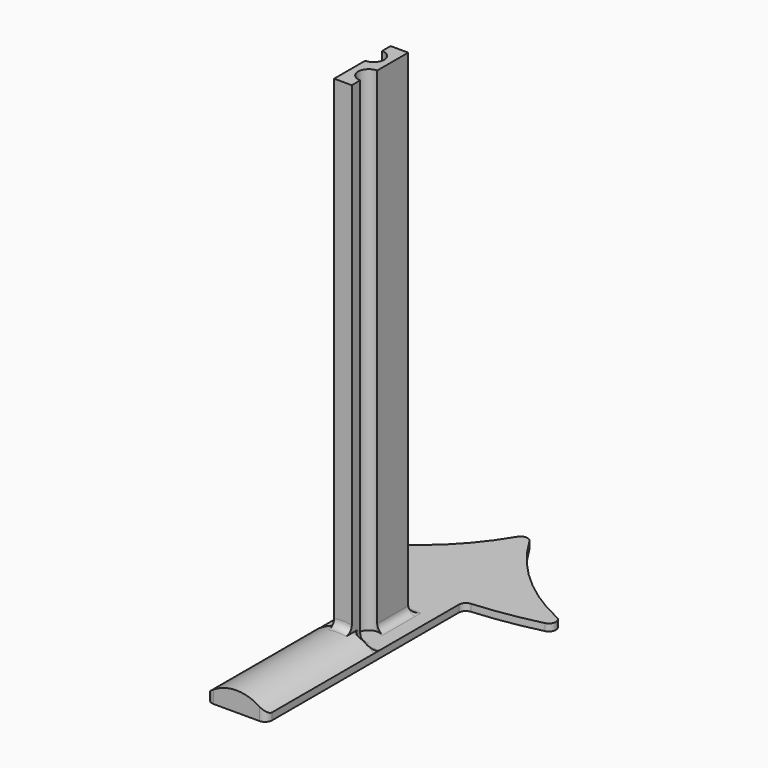
from build123d import *

# Parameters (mm, degrees)
F1_DEPTH      = 2
F3_DEPTH      = 140
F5_DEPTH      = 38
F6_S2_W       = 2
F6_S2_H       = 2
F6_T3_DEPTH   = 2
F6_S7_W       = 2
F6_S7_H       = 2
F6_T8_DEPTH   = 2
F6_T13_DEPTH  = 16
F6_S14_R      = 3
F6_T15_DEPTH  = 10
F6_T18_DEPTH  = 8
F6_S19_R      = 3
F6_T20_DEPTH  = 6
F6_T23_DEPTH  = 5
F6_T26_DEPTH  = 2
F6_T29_DEPTH  = 2
F6_T32_DEPTH  = 6.2698148841
F6_S33_R      = 12
F6_T34_DEPTH  = 5
F6_T37_DEPTH  = 4.0036432176
F6_S38_R      = 12
F6_T39_DEPTH  = 4
F6_T42_DEPTH  = 6.2698148841
F6_S43_R      = 12
F6_T44_DEPTH  = 5
F6_T47_DEPTH  = 4.0036432176
F6_S48_R      = 12
F6_T49_DEPTH  = 4
F6_T52_DEPTH  = 13.7211477996
F6_S53_R      = 3
F6_T54_DEPTH  = 9
F6_T57_DEPTH  = 5.7211477996
F6_S58_R      = 3
F6_T59_DEPTH  = 5
F6_T62_ANGLE  = 71.7972504735
F6_T68_DEPTH  = 21
F6_T72_DEPTH  = 10
F6_T78_DEPTH  = 10
F6_T82_DEPTH  = 13
F6_T88_DEPTH  = 12
F6_T91_DEPTH  = 12
F6_T94_DEPTH  = 32.0377713688
F6_T97_DEPTH  = 32.0377713688
F6_T100_DEPTH = 19.7312172526


# Not quite as in the source:
# - a fillet or chamfer that OpenCascade refuses, or shapes differently, is made with other operations: its cross-section is extruded or revolved along the edge and cut away or added


with BuildPart() as f1:
    # F0 (on Top) → F1 (new body)
    with BuildSketch(Plane.XY):
        with BuildLine():
            ThreePointArc((-34.7443990516, -30.0072931229), (-21.7619757905, -33.1321767709), (-8.5036432176, -34.7211477996))
            Line((-8.5036432176, -34.7211477996), (-8.5036432176, -104.7211477996))
            Line((-8.5036432176, -104.7211477996), (0, -104.7211477996))
            Line((0, -104.7211477996), (8.5036432176, -104.7211477996))
            Line((8.5036432176, -104.7211477996), (8.5036432176, -34.7211477996))
            ThreePointArc((8.5036432176, -34.7211477996), (21.7619757905, -33.1321767709), (34.7443990516, -30.0072931229))
            ThreePointArc((34.7443990516, -30.0072931229), (14.4817817228, -18.350360614), (0, 0))
            ThreePointArc((0, 0), (-14.4817817228, -18.350360614), (-34.7443990516, -30.0072931229))
        make_face()
    extrude(amount=F1_DEPTH)

    # F2 (on face) → F3 (join)
    with BuildSketch(Plane.XY.offset(2)):
        with BuildLine():
            Line((-2.5, -67), (2.5, -67))
            Line((2.5, -67), (2.5, -64))
            ThreePointArc((2.5, -64), (-0.5, -61), (2.5, -58))
            Line((2.5, -58), (2.5, -47))
            Line((2.5, -47), (-2.5, -47))
            Line((-2.5, -47), (-2.5, -50))
            ThreePointArc((-2.5, -50), (0.5, -53), (-2.5, -56))
            Line((-2.5, -56), (-2.5, -67))
        make_face()
    extrude(amount=F3_DEPTH)

    # F4 (on face) → F5 (join)
    with BuildSketch(Plane.XZ.offset(104.7211477996)):
        with BuildLine():
            ThreePointArc((8.5036432176, 2), (0, 5.5331202898), (-8.5036432176, 2))
            Line((-8.5036432176, 2), (8.5036432176, 2))
        make_face()
    extrude(amount=-F5_DEPTH)

    # F6: fillet of radius 2 on 17 edges, made by hand


with BuildPart() as f6_tool1:
    # F6_s2 → F6_t3 (new body)
    with BuildSketch(Plane.XZ.offset(64.7211477996)):
        with Locations((3.5, 3)):
            Rectangle(F6_S2_W, F6_S2_H)
    extrude(amount=F6_T3_DEPTH)

    # F6_s4 → F6_t5 (revolve, cut)
    with BuildSketch(Plane(origin=(4.5, -64.7211477996, 4), x_dir=(0.7071067812, 0, 0.7071067812), z_dir=(0.7071067812, 0, -0.7071067812))):
        with BuildLine():
            ThreePointArc((0, -2), (2, 0), (0, 2))
            Line((0, 2), (0, -2))
        make_face()
    revolve(axis=Axis((4.5, -64.7211477996, 4), (0, -1, 0)), mode=Mode.SUBTRACT)


with BuildPart() as f6_tool6:
    # F6_s7 → F6_t8 (new body)
    with BuildSketch(Plane.YZ.offset(-4.5)):
        with Locations((-65.7211477996, 3)):
            Rectangle(F6_S7_W, F6_S7_H)
    extrude(amount=F6_T8_DEPTH)

    # F6_s9 → F6_t10 (revolve, cut)
    with BuildSketch(Plane(origin=(-4.5, -64.7211477996, 4), x_dir=(0, 0.7071067812, 0.7071067812), z_dir=(0, 0.7071067812, -0.7071067812))):
        with BuildLine():
            ThreePointArc((0, -2), (2, 0), (0, 2))
            Line((0, 2), (0, -2))
        make_face()
    revolve(axis=Axis((-4.5, -64.7211477996, 4), (1, 0, 0)), mode=Mode.SUBTRACT)


with BuildPart() as f6_tool11:
    # F6_s12 → F6_t13 (new body)
    with BuildSketch(Plane.XZ.offset(63)):
        with BuildLine():
            ThreePointArc((4.5, 2), (3.0857864376, 2.5857864376), (2.5, 4))
            Line((2.5, 4), (2.5, 2))
            Line((2.5, 2), (4.5, 2))
        make_face()
    extrude(amount=-F6_T13_DEPTH)

    # F6_s14 → F6_t15 (cut, symmetric)
    with BuildSketch(Plane.XY.offset(3)):
        with Locations((2.5, -61)):
            Circle(F6_S14_R)
    extrude(amount=F6_T15_DEPTH, both=True, mode=Mode.SUBTRACT)


with BuildPart() as f6_tool16:
    # F6_s17 → F6_t18 (new body)
    with BuildSketch(Plane.XZ.offset(47)):
        with BuildLine():
            ThreePointArc((-4.5, 2), (-3.0857864376, 2.5857864376), (-2.5, 4))
            Line((-2.5, 4), (-2.5, 2))
            Line((-2.5, 2), (-4.5, 2))
        make_face()
    extrude(amount=F6_T18_DEPTH)

    # F6_s19 → F6_t20 (cut, symmetric)
    with BuildSketch(Plane.XY.offset(3)):
        with Locations((-2.5, -53)):
            Circle(F6_S19_R)
    extrude(amount=F6_T20_DEPTH, both=True, mode=Mode.SUBTRACT)


with BuildPart() as f6_tool21:
    # F6_s22 → F6_t23 (new body)
    with BuildSketch(Plane.YZ.offset(2.5)):
        with BuildLine():
            ThreePointArc((-45, 2), (-46.4142135624, 2.5857864376), (-47, 4))
            Line((-47, 4), (-47, 2))
            Line((-47, 2), (-45, 2))
        make_face()
    extrude(amount=-F6_T23_DEPTH)


with BuildPart() as f6_tool24:
    # F6_s25 → F6_t26 (new body)
    with BuildSketch(Plane.XY):
        with BuildLine():
            ThreePointArc((-10.349778168, -34.5937272007), (-9.0360380086, -35.2290743164), (-8.5036432176, -36.5877998039))
            Line((-8.5036432176, -36.5877998039), (-8.5036432176, -34.7211477996))
            ThreePointArc((-8.5036432176, -34.7211477996), (-9.4269686479, -34.6611748852), (-10.349778168, -34.5937272007))
        make_face()
    extrude(amount=F6_T26_DEPTH)


with BuildPart() as f6_tool27:
    # F6_s28 → F6_t29 (new body)
    with BuildSketch(Plane.XY):
        with BuildLine():
            ThreePointArc((10.349778168, -34.5937272007), (9.0360380086, -35.2290743164), (8.5036432176, -36.5877998039))
            Line((8.5036432176, -36.5877998039), (8.5036432176, -34.7211477996))
            ThreePointArc((8.5036432176, -34.7211477996), (9.4269686479, -34.6611748852), (10.349778168, -34.5937272007))
        make_face()
    extrude(amount=F6_T29_DEPTH)


with BuildPart() as f6_tool30:
    # F6_s31 → F6_t32 (new body)
    with BuildSketch(Plane.XY.offset(4)):
        with BuildLine():
            ThreePointArc((4.5, -66.7211477996), (3.0857864376, -66.135361362), (2.5, -64.7211477996))
            Line((2.5, -64.7211477996), (2.5, -66.7211477996))
            Line((2.5, -66.7211477996), (4.5, -66.7211477996))
        make_face()
    extrude(amount=F6_T32_DEPTH)

    # F6_s33 → F6_t34 (intersect, symmetric)
    with BuildSketch(Plane.XZ.offset(65.7)):
        with Locations((0, -6.4668797102)):
            Circle(F6_S33_R)
    extrude(amount=F6_T34_DEPTH, both=True, mode=Mode.INTERSECT)


with BuildPart() as f6_tool35:
    # F6_s36 → F6_t37 (new body)
    with BuildSketch(Plane.YZ.offset(4.5)):
        with BuildLine():
            ThreePointArc((-64.7211477996, 2), (-66.135361362, 2.5857864376), (-66.7211477996, 4))
            Line((-66.7211477996, 4), (-66.7211477996, 2))
            Line((-66.7211477996, 2), (-64.7211477996, 2))
        make_face()
    extrude(amount=F6_T37_DEPTH)

    # F6_s38 → F6_t39 (intersect, symmetric)
    with BuildSketch(Plane.XZ.offset(65.7)):
        with Locations((0, -6.4668797102)):
            Circle(F6_S38_R)
    extrude(amount=F6_T39_DEPTH, both=True, mode=Mode.INTERSECT)


with BuildPart() as f6_tool40:
    # F6_s41 → F6_t42 (new body)
    with BuildSketch(Plane.XY.offset(10.2698148841)):
        with BuildLine():
            ThreePointArc((-2.5, -64.7211477996), (-3.0857864376, -66.135361362), (-4.5, -66.7211477996))
            Line((-4.5, -66.7211477996), (-2.5, -66.7211477996))
            Line((-2.5, -66.7211477996), (-2.5, -64.7211477996))
        make_face()
    extrude(amount=-F6_T42_DEPTH)

    # F6_s43 → F6_t44 (intersect, symmetric)
    with BuildSketch(Plane.XZ.offset(65.7)):
        with Locations((0, -6.4668797102)):
            Circle(F6_S43_R)
    extrude(amount=F6_T44_DEPTH, both=True, mode=Mode.INTERSECT)


with BuildPart() as f6_tool45:
    # F6_s46 → F6_t47 (new body)
    with BuildSketch(Plane.YZ.offset(-8.5036432176)):
        with BuildLine():
            ThreePointArc((-64.7211477996, 2), (-66.135361362, 2.5857864376), (-66.7211477996, 4))
            Line((-66.7211477996, 4), (-66.7211477996, 2))
            Line((-66.7211477996, 2), (-64.7211477996, 2))
        make_face()
    extrude(amount=F6_T47_DEPTH)

    # F6_s48 → F6_t49 (intersect, symmetric)
    with BuildSketch(Plane.XZ.offset(65.7)):
        with Locations((0, -6.4668797102)):
            Circle(F6_S48_R)
    extrude(amount=F6_T49_DEPTH, both=True, mode=Mode.INTERSECT)


with BuildPart() as f6_tool50:
    # F6_s51 → F6_t52 (new body)
    with BuildSketch(Plane.XZ.offset(51)):
        with BuildLine():
            ThreePointArc((-4.5, 2), (-3.0857864376, 2.5857864376), (-2.5, 4))
            Line((-2.5, 4), (-2.5, 2))
            Line((-2.5, 2), (-4.5, 2))
        make_face()
    extrude(amount=F6_T52_DEPTH)

    # F6_s53 → F6_t54 (cut, symmetric)
    with BuildSketch(Plane.XY.offset(3)):
        with Locations((-2.5, -53)):
            Circle(F6_S53_R)
    extrude(amount=F6_T54_DEPTH, both=True, mode=Mode.SUBTRACT)


with BuildPart() as f6_tool55:
    # F6_s56 → F6_t57 (new body)
    with BuildSketch(Plane.XZ.offset(64.7211477996)):
        with BuildLine():
            ThreePointArc((4.5, 2), (3.0857864376, 2.5857864376), (2.5, 4))
            Line((2.5, 4), (2.5, 2))
            Line((2.5, 2), (4.5, 2))
        make_face()
    extrude(amount=-F6_T57_DEPTH)

    # F6_s58 → F6_t59 (cut, symmetric)
    with BuildSketch(Plane.XY.offset(3)):
        with Locations((2.5, -61)):
            Circle(F6_S58_R)
    extrude(amount=F6_T59_DEPTH, both=True, mode=Mode.SUBTRACT)


with BuildPart() as f6_tool60:
    # F6_s61 → F6_t62 (revolve)
    with BuildSketch(Plane(origin=(3.0716290249, 0, -2.2233762781), x_dir=(0, 1, 0), z_dir=(0.8100557097, 0, -0.5863529203))):
        with BuildLine():
            ThreePointArc((-69, 6.7614671667), (-67.5857864376, 7.3472536043), (-67, 8.7614671667))
            Line((-67, 8.7614671667), (-67, 6.7614671667))
            Line((-67, 6.7614671667), (-69, 6.7614671667))
        make_face()
    revolve(axis=Axis((0, -67, -6.4668797102), (0, -1, 0)), revolution_arc=F6_T62_ANGLE)

    split(bisect_by=Plane.YZ.offset(2.5), keep=Keep.BOTTOM)

    split(bisect_by=Plane.YZ.offset(-2.5), keep=Keep.TOP)


with BuildPart() as f6_tool66:
    # F6_s67 → F6_t68 (new body)
    with BuildSketch(Plane.XZ.offset(63)):
        with BuildLine():
            ThreePointArc((4.5, 2), (3.0857864376, 2.5857864376), (2.5, 4))
            Line((2.5, 4), (2.5, 2))
            Line((2.5, 2), (4.5, 2))
        make_face()
    extrude(amount=-F6_T68_DEPTH)

    split(bisect_by=Plane.XZ.offset(47), keep=Keep.BOTTOM)


with BuildPart() as f6_tool70:
    # F6_s71 → F6_t72 (new body)
    with BuildSketch(Plane.YZ.offset(7.5)):
        with BuildLine():
            ThreePointArc((-45, 2), (-46.4142135624, 2.5857864376), (-47, 4))
            Line((-47, 4), (-47, 2))
            Line((-47, 2), (-45, 2))
        make_face()
    extrude(amount=-F6_T72_DEPTH)

    split(bisect_by=Plane.YZ.offset(2.5), keep=Keep.TOP)


with BuildPart() as f6_tool66_1:
    add(f6_tool66.part)

    # F6_t74: intersect F6_tool70
    add(f6_tool70.part, mode=Mode.INTERSECT)


with BuildPart() as f6_tool76:
    # F6_s77 → F6_t78 (new body)
    with BuildSketch(Plane.YZ.offset(2.5)):
        with BuildLine():
            ThreePointArc((-45, 2), (-46.4142135624, 2.5857864376), (-47, 4))
            Line((-47, 4), (-47, 2))
            Line((-47, 2), (-45, 2))
        make_face()
    extrude(amount=-F6_T78_DEPTH)

    split(bisect_by=Plane.YZ.offset(-2.5), keep=Keep.BOTTOM)


with BuildPart() as f6_tool80:
    # F6_s81 → F6_t82 (new body)
    with BuildSketch(Plane.XZ.offset(42)):
        with BuildLine():
            ThreePointArc((-4.5, 2), (-3.0857864376, 2.5857864376), (-2.5, 4))
            Line((-2.5, 4), (-2.5, 2))
            Line((-2.5, 2), (-4.5, 2))
        make_face()
    extrude(amount=F6_T82_DEPTH)

    split(bisect_by=Plane.XZ.offset(47), keep=Keep.BOTTOM)


with BuildPart() as f6_tool76_1:
    add(f6_tool76.part)

    # F6_t84: intersect F6_tool80
    add(f6_tool80.part, mode=Mode.INTERSECT)


with BuildPart() as f1_1:
    add(f1.part)

    # F6_t85: union F6_tool1, F6_tool6, F6_tool11, F6_tool16, F6_tool21, F6_tool24, F6_tool27, F6_tool30, F6_tool35, F6_tool40, F6_tool45, F6_tool50, F6_tool55, F6_tool60, F6_tool66, F6_tool76
    add([f6_tool1.part, f6_tool6.part, f6_tool11.part, f6_tool16.part, f6_tool21.part, f6_tool24.part, f6_tool27.part, f6_tool30.part, f6_tool35.part, f6_tool40.part, f6_tool45.part, f6_tool50.part, f6_tool55.part, f6_tool60.part, f6_tool66_1.part, f6_tool76_1.part])


with BuildPart() as f6_tool86:
    # F6_s87 → F6_t88 (new body)
    with BuildSketch(Plane.XY.offset(-5)):
        with BuildLine():
            ThreePointArc((-6.5036432176, -104.7211477996), (-7.91785678, -104.135361362), (-8.5036432176, -102.7211477996))
            Line((-8.5036432176, -102.7211477996), (-8.5036432176, -104.7211477996))
            Line((-8.5036432176, -104.7211477996), (-6.5036432176, -104.7211477996))
        make_face()
    extrude(amount=F6_T88_DEPTH)


with BuildPart() as f6_tool89:
    # F6_s90 → F6_t91 (new body)
    with BuildSketch(Plane.XY.offset(-5)):
        with BuildLine():
            ThreePointArc((8.5036432176, -102.7211477996), (7.91785678, -104.135361362), (6.5036432176, -104.7211477996))
            Line((6.5036432176, -104.7211477996), (8.5036432176, -104.7211477996))
            Line((8.5036432176, -104.7211477996), (8.5036432176, -102.7211477996))
        make_face()
    extrude(amount=F6_T91_DEPTH)


with BuildPart() as f6_tool92:
    # F6_s93 → F6_t94 (new body)
    with BuildSketch(Plane.XY.offset(-15.0188856844)):
        with BuildLine():
            ThreePointArc((28.9519071991, -31.6003237222), (30.4639347839, -29.8429196175), (29.300045112, -27.8379115286))
            ThreePointArc((29.300045112, -27.8379115286), (31.9964862312, -28.987189893), (34.7443990516, -30.0072931229))
            ThreePointArc((34.7443990516, -30.0072931229), (31.8586243798, -30.8418834327), (28.9519071991, -31.6003237222))
        make_face()
    extrude(amount=F6_T94_DEPTH)


with BuildPart() as f6_tool95:
    # F6_s96 → F6_t97 (new body)
    with BuildSketch(Plane.XY.offset(-15.0188856844)):
        with BuildLine():
            ThreePointArc((-29.300045112, -27.8379115286), (-30.4639347839, -29.8429196175), (-28.9519071991, -31.6003237222))
            ThreePointArc((-28.9519071991, -31.6003237222), (-31.8586243798, -30.8418834327), (-34.7443990516, -30.0072931229))
            ThreePointArc((-34.7443990516, -30.0072931229), (-31.9964862312, -28.987189893), (-29.300045112, -27.8379115286))
        make_face()
    extrude(amount=F6_T97_DEPTH)


with BuildPart() as f6_tool98:
    # F6_s99 → F6_t100 (new body)
    with BuildSketch(Plane.XY.offset(-8.8656086263)):
        with BuildLine():
            ThreePointArc((-1.7203370706, -3.1010132173), (0, -2.1210330032), (1.7203370706, -3.1010132173))
            ThreePointArc((1.7203370706, -3.1010132173), (0.8379162788, -1.5628514066), (0, 0))
            ThreePointArc((0, 0), (-0.8379162788, -1.5628514066), (-1.7203370706, -3.1010132173))
        make_face()
    extrude(amount=F6_T100_DEPTH)


with BuildPart() as f1_2:
    add(f1_1.part)

    # F6_t101: cut F6_tool86, F6_tool89, F6_tool92, F6_tool95, F6_tool98
    add([f6_tool86.part, f6_tool89.part, f6_tool92.part, f6_tool95.part, f6_tool98.part], mode=Mode.SUBTRACT)


solid = f1_2.part
